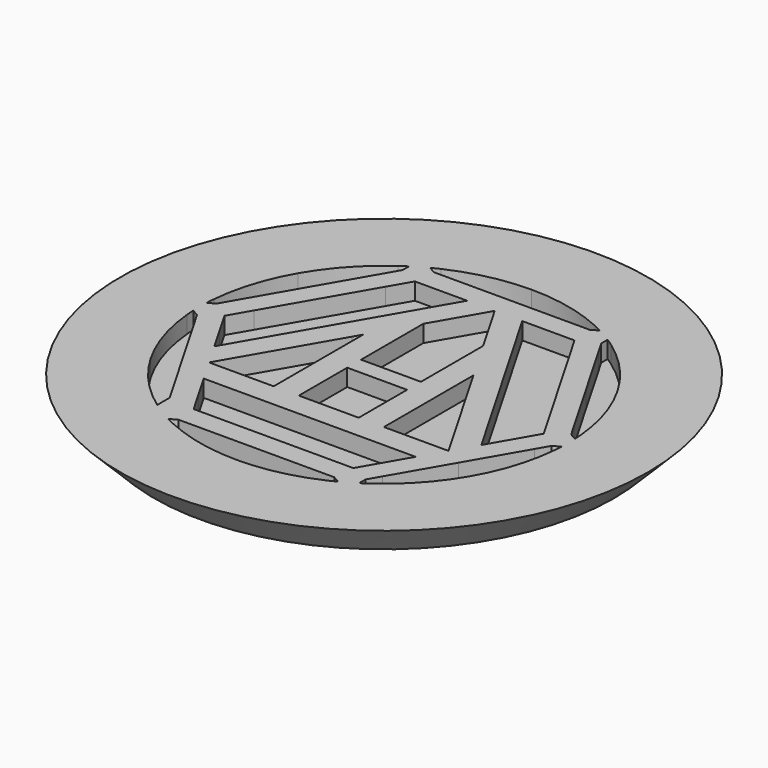
from build123d import *

# Parameters (mm, degrees)
F0_R     = 32
F1_DEPTH = 4
F3_R     = 5.5
F3_R_2   = 4.025
F4_DEPTH = 1.5
F5_DEPTH = 6.5
F7_DEPTH = 2
F8_R     = 2


# Not quite as in the source:
# - a fillet or chamfer that OpenCascade refuses, or shapes differently, is made with other operations: its cross-section is extruded or revolved along the edge and cut away or added


with BuildPart() as f1:
    # F0 (on Top) → F1 (new body)
    with BuildSketch(Plane.XY):
        Circle(F0_R)
    extrude(amount=F1_DEPTH)

    # F2: chamfer of 5 on 1 edges, made by hand

    # F2_s1 → F2_t2 (revolve, cut)
    with BuildSketch(Plane.XZ):
        Polygon((32, 5), (27, 0), (32, 0), align=None)
    revolve(axis=Axis((0, 0, 0), (0, 0, 1)), mode=Mode.SUBTRACT)

    # F3 (on face) → F4 (join)
    with BuildSketch(Plane(origin=(0, 0, 0), x_dir=(1, 0, 0), z_dir=(0, 0, -1))):
        Circle(F3_R)
        Circle(F3_R_2, mode=Mode.SUBTRACT)
    extrude(amount=F4_DEPTH)

    # F3 (on face) → F5 (join)
    with BuildSketch(Plane(origin=(0, 0, 0), x_dir=(1, 0, 0), z_dir=(0, 0, -1))):
        Circle(F3_R_2)
    extrude(amount=F5_DEPTH)

    # F6 (on face) → F7 (cut)
    with BuildSketch(Plane.XY.offset(4)):
        with BuildLine():
            Line((16.237976321, -9.375), (18.75, -10.8253175473))
            ThreePointArc((18.75, -10.8253175473), (20.6335015486, -6.5580952909), (21.5593108924, -1.9864827825))
            Line((21.5593108924, -1.9864827825), (19.9759526419, -2.9006350946))
            Line((19.9759526419, -2.9006350946), (16.237976321, -9.375))
        make_face()
        with BuildLine():
            ThreePointArc((12.5, -17.6776695297), (15.9962278967, -14.5900888646), (18.75, -10.8253175473))
            Line((18.75, -10.8253175473), (16.237976321, -9.375))
            Line((16.237976321, -9.375), (12.5, -15.8493649054))
            Line((12.5, -15.8493649054), (12.5, -17.6776695297))
        make_face()
        with BuildLine():
            ThreePointArc((21.5593108924, 1.9864827825), (20.6335020609, 6.5580936791), (18.7500016913, 10.8253146179))
            ThreePointArc((18.7500016913, 10.8253146179), (15.9962290364, 14.590087615), (12.5, 17.6776695297))
            Line((12.5, 17.6776695297), (12.5, 15.8493649054))
            Line((12.5, 15.8493649054), (16.2379763781, 9.3749999011))
            Line((16.2379763781, 9.3749999011), (19.9759526419, 2.9006350946))
            Line((19.9759526419, 2.9006350946), (21.5593108924, 1.9864827825))
        make_face()
        with BuildLine():
            ThreePointArc((9.0593108924, 19.6641523121), (4.6372736512, 21.1481841557), (-1.3e-09, 21.6506350946))
            ThreePointArc((-1.3e-09, 21.6506350946), (-4.6372736525, 21.1481841554), (-9.0593108924, 19.6641523121))
            Line((-9.0593108924, 19.6641523121), (-7.4759526419, 18.75))
            Line((-7.4759526419, 18.75), (-3.65e-08, 18.75))
            Line((-3.65e-08, 18.75), (7.4759526419, 18.75))
            Line((7.4759526419, 18.75), (9.0593108924, 19.6641523121))
        make_face()
        with BuildLine():
            ThreePointArc((-9.0593108924, -19.6641523121), (-4.6372736547, -21.1481841549), (-5.7e-09, -21.6506350946))
            ThreePointArc((-5.7e-09, -21.6506350946), (4.6372736491, -21.1481841562), (9.0593108924, -19.6641523121))
            Line((9.0593108924, -19.6641523121), (7.4759526419, -18.75))
            Line((7.4759526419, -18.75), (0, -18.75))
            Line((0, -18.75), (-7.4759526419, -18.75))
            Line((-7.4759526419, -18.75), (-9.0593108924, -19.6641523121))
        make_face()
        with BuildLine():
            ThreePointArc((11.6626587737, -18.2409536573), (12.0846117855, -17.9641909919), (12.5, -17.6776695297))
            Line((12.5, -17.6776695297), (12.5, -15.8493649054))
            Line((12.5, -15.8493649054), (11.6626587737, -17.2996824527))
            Line((11.6626587737, -17.2996824527), (11.6626587737, -18.2409536573))
        make_face()
        with BuildLine():
            Line((19.9759526419, -2.9006350946), (21.5593108924, -1.9864827825))
            ThreePointArc((21.5593108924, -1.9864827825), (21.5997516502, -1.4834853051), (21.6284586433, -0.979681945))
            Line((21.6284586433, -0.979681945), (20.8132938683, -1.4503175473))
            Line((20.8132938683, -1.4503175473), (19.9759526419, -2.9006350946))
        make_face()
        with BuildLine():
            ThreePointArc((21.6284586433, 0.979681945), (21.5997516502, 1.4834853051), (21.5593108924, 1.9864827825))
            Line((21.5593108924, 1.9864827825), (19.9759526419, 2.9006350946))
            Line((19.9759526419, 2.9006350946), (20.8132938683, 1.4503175473))
            Line((20.8132938683, 1.4503175473), (21.6284586433, 0.979681945))
        make_face()
        with BuildLine():
            Line((12.5, 15.8493649054), (12.5, 17.6776695297))
            ThreePointArc((12.5, 17.6776695297), (12.0846117855, 17.9641909919), (11.6626587737, 18.2409536573))
            Line((11.6626587737, 18.2409536573), (11.6626587737, 17.2996824527))
            Line((11.6626587737, 17.2996824527), (12.5, 15.8493649054))
        make_face()
        with BuildLine():
            ThreePointArc((-12.5, 17.6776695297), (-15.9962290427, 14.5900876082), (-18.7500017006, 10.8253146018))
            ThreePointArc((-18.7500017006, 10.8253146018), (-20.6335020637, 6.5580936703), (-21.5593108924, 1.9864827825))
            Line((-21.5593108924, 1.9864827825), (-19.9759526419, 2.9006350946))
            Line((-19.9759526419, 2.9006350946), (-16.2379762959, 9.3750000433))
            Line((-16.2379762959, 9.3750000433), (-12.5, 15.8493649054))
            Line((-12.5, 15.8493649054), (-12.5, 17.6776695297))
        make_face()
        with BuildLine():
            ThreePointArc((9.9657998697, 19.2206356023), (9.5151398647, 19.447676297), (9.0593108924, 19.6641523121))
            Line((9.0593108924, 19.6641523121), (7.4759526419, 18.75))
            Line((7.4759526419, 18.75), (9.1506350946, 18.75))
            Line((9.1506350946, 18.75), (9.9657998697, 19.2206356023))
        make_face()
        with BuildLine():
            Line((-7.4759526419, 18.75), (-9.0593108924, 19.6641523121))
            ThreePointArc((-9.0593108924, 19.6641523121), (-9.5151398647, 19.447676297), (-9.9657998697, 19.2206356023))
            Line((-9.9657998697, 19.2206356023), (-9.1506350946, 18.75))
            Line((-9.1506350946, 18.75), (-7.4759526419, 18.75))
        make_face()
        with BuildLine():
            Line((-16.237976321, -9.375), (-18.75, -10.8253175473))
            ThreePointArc((-18.75, -10.8253175473), (-15.9962278967, -14.5900888646), (-12.5, -17.6776695297))
            Line((-12.5, -17.6776695297), (-12.5, -15.8493649054))
            Line((-12.5, -15.8493649054), (-16.237976321, -9.375))
        make_face()
        with BuildLine():
            ThreePointArc((-21.5593108924, -1.9864827825), (-20.6335015486, -6.5580952909), (-18.75, -10.8253175473))
            Line((-18.75, -10.8253175473), (-16.237976321, -9.375))
            Line((-16.237976321, -9.375), (-19.9759526419, -2.9006350946))
            Line((-19.9759526419, -2.9006350946), (-21.5593108924, -1.9864827825))
        make_face()
        with BuildLine():
            ThreePointArc((-9.9657998697, -19.2206356023), (-9.5151398647, -19.447676297), (-9.0593108924, -19.6641523121))
            Line((-9.0593108924, -19.6641523121), (-7.4759526419, -18.75))
            Line((-7.4759526419, -18.75), (-9.1506350946, -18.75))
            Line((-9.1506350946, -18.75), (-9.9657998697, -19.2206356023))
        make_face()
        with BuildLine():
            Line((7.4759526419, -18.75), (9.0593108924, -19.6641523121))
            ThreePointArc((9.0593108924, -19.6641523121), (9.5151398647, -19.447676297), (9.9657998697, -19.2206356023))
            Line((9.9657998697, -19.2206356023), (9.1506350946, -18.75))
            Line((9.1506350946, -18.75), (7.4759526419, -18.75))
        make_face()
        Polygon((6.4743649054, -16.237976321), (9.375, -16.237976321), (10.8253175473, -13.7259526419), align=None)
        Polygon((17.2996824527, -2.512023679), (18.75, 0), (17.2996824527, 2.512023679), align=None)
        with BuildLine():
            ThreePointArc((-11.6626587737, 18.2409536573), (-12.0846117855, 17.9641909919), (-12.5, 17.6776695297))
            Line((-12.5, 17.6776695297), (-12.5, 15.8493649054))
            Line((-12.5, 15.8493649054), (-11.6626587737, 17.2996824527))
            Line((-11.6626587737, 17.2996824527), (-11.6626587737, 18.2409536573))
        make_face()
        with BuildLine():
            Line((-19.9759526419, 2.9006350946), (-21.5593108924, 1.9864827825))
            ThreePointArc((-21.5593108924, 1.9864827825), (-21.5997516502, 1.4834853051), (-21.6284586433, 0.979681945))
            Line((-21.6284586433, 0.979681945), (-20.8132938683, 1.4503175473))
            Line((-20.8132938683, 1.4503175473), (-19.9759526419, 2.9006350946))
        make_face()
        with BuildLine():
            ThreePointArc((-21.6284586433, -0.979681945), (-21.5997516502, -1.4834853051), (-21.5593108924, -1.9864827825))
            Line((-21.5593108924, -1.9864827825), (-19.9759526419, -2.9006350946))
            Line((-19.9759526419, -2.9006350946), (-20.8132938683, -1.4503175473))
            Line((-20.8132938683, -1.4503175473), (-21.6284586433, -0.979681945))
        make_face()
        Polygon((0, -16.237976321), (6.4743649054, -16.237976321), (10.8253175473, -13.7259526419), (12.4439087737, -10.9224704012), (-12.4439087737, -10.9224704012), (-10.8253175473, -13.7259526419), (-6.4743649054, -16.237976321), align=None)
        Polygon((15.6810912263, -5.3155059198), (17.2996824527, -2.512023679), (17.2996824527, 2.512023679), (10.8253175473, 13.7259526419), (6.4743649054, 16.237976321), (3.2371824527, 16.237976321), align=None)
        Polygon((-17.2996824527, 2.512023679), (-18.75, 0), (-17.2996824527, -2.512023679), align=None)
        Polygon((-10.8253175473, -13.7259526419), (-9.375, -16.237976321), (-6.4743649054, -16.237976321), align=None)
        Polygon((-7.03125, 4.0594940802), (-14.0625, -8.1189881605), (-6.4743649054, -8.1189881605), (-6.4743649054, 5.0240473581), align=None)
        Polygon((10.8253175473, 13.7259526419), (9.375, 16.237976321), (6.4743649054, 16.237976321), align=None)
        Polygon((-6.4743649054, 16.237976321), (-9.375, 16.237976321), (-10.8253175473, 13.7259526419), align=None)
        Polygon((-10.8253175473, 13.7259526419), (-17.2996824527, 2.512023679), (-17.2996824527, -2.512023679), (-15.6810912263, -5.3155059198), (-3.2371824527, 16.237976321), (-6.4743649054, 16.237976321), align=None)
        Polygon((6.4743649054, -8.1189881605), (14.0625, -8.1189881605), (7.03125, 4.0594940802), (6.4743649054, 5.0240473581), align=None)
        Polygon((-3.515625, -4.0594940802), (-3.515625, -8.1189881605), (3.515625, -8.1189881605), (3.515625, -1.0148735201), (0, -1.0148735201), (-3.515625, -1.0148735201), (-3.515625, -2.0297470401), align=None)
        Polygon((3.515625, 10.1487352006), (0, 16.237976321), (-3.515625, 10.1487352006), (-3.515625, 1.0148735201), (0, 1.0148735201), (3.515625, 1.0148735201), align=None)
    extrude(amount=-F7_DEPTH, mode=Mode.SUBTRACT)

    # F8
    f8_edges = [f1.edges().sort_by_distance(p)[0] for p in [
        (-4.025, 0, -6.5),
    ]]
    fillet(f8_edges, radius=F8_R)


solid = f1.part
